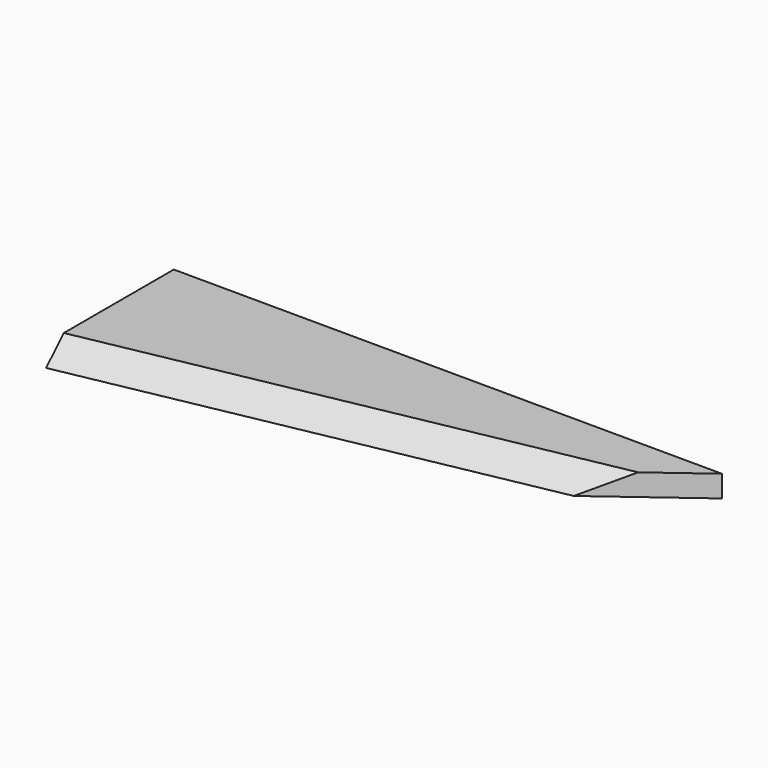
from build123d import *

# Parameters (mm, degrees)
F1_DEPTH    = 2.54
F2_T1_DEPTH = 75.625199713


# Not quite as in the source:
# - a fillet or chamfer that OpenCascade refuses, or shapes differently, is made with other operations: its cross-section is extruded or revolved along the edge and cut away or added


with BuildPart() as f1:
    # F0 (on Top) → F1 (new body)
    with BuildSketch(Plane.XY):
        Polygon((21.8819305301, 6.1752684414), (-42.2871634364, 6.4437580295), (-42.2871634364, -14.766946435), (6.30951114, -5.369798746), align=None)
    extrude(amount=F1_DEPTH)

    # F2: chamfer of 5.08 on 1 edges, made by hand

    # F2_s2 → F2_t1 (cut)
    with BuildSketch(Plane(origin=(-56.3420622243, -10.8948746893, 0), x_dir=(0, 0, 1), z_dir=(0.9818124778, 0.1898532551, 0))):
        Polygon((-2.54, 6.4700166401), (2.54, 1.3900166401), (2.54, 6.4700166401), align=None)
    extrude(amount=F2_T1_DEPTH, mode=Mode.SUBTRACT)


solid = f1.part
